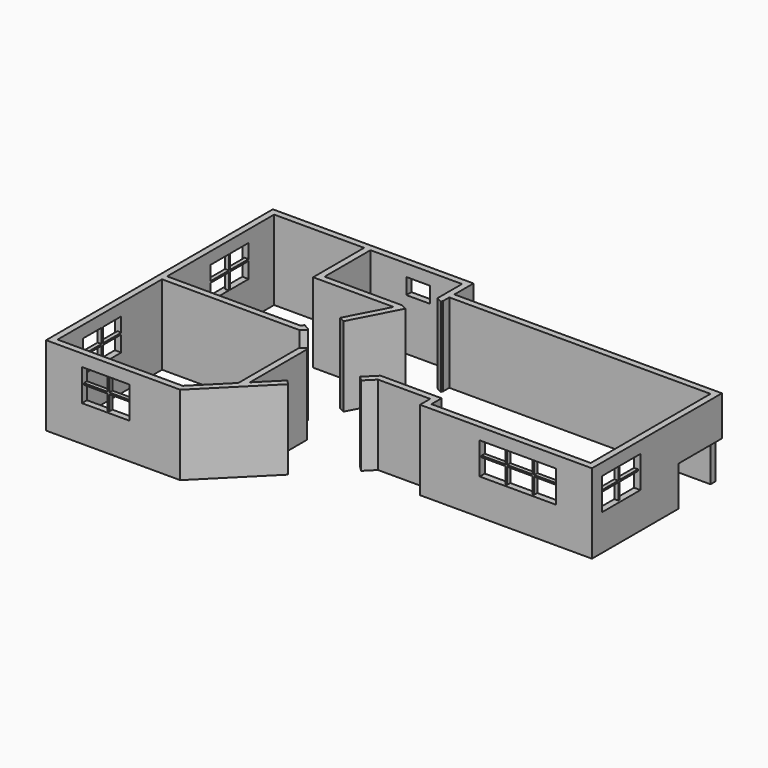
from build123d import *

# Parameters (mm, degrees)
F1_DEPTH  = 2540
F2_W      = 736.6
F2_H      = 457.2
F2_H_2    = 508
F3_DEPTH  = 203.2
F4_W      = 1524
F4_H      = 1016
F5_DEPTH  = 76.2
F6_W      = 762
F6_H      = 482.6
F6_W_2    = 711.2
F7_DEPTH  = 203.2
F8_W      = 1524
F8_H      = 1016
F9_DEPTH  = 76.2
F10_W     = 762
F10_H     = 457.2
F10_W_2   = 812.8
F10_H_2   = 508
F11_DEPTH = 203.2
F12_W     = 2438.4
F12_H     = 1016
F13_DEPTH = 76.2
F14_W     = 762
F14_H     = 508
F15_DEPTH = 203.2
F16_W     = 203.2
F16_H     = 1270
F16_W_2   = 1524
F17_DEPTH = 203.2
F18_W     = 736.6
F18_H     = 508
F19_DEPTH = 203.2
F20_W     = 1524
F20_H     = 1016
F21_DEPTH = 76.2


# Not quite as in the source:
# - ends of sketch curves that miss each other by under 0.0002 mm in the source are joined


with BuildPart() as f1:
    # F0 (on Top) → F1 (new body)
    with BuildSketch(Plane.XY):
        Polygon((0, 10668), (0, 1625.6), (4279.6544454742, 1625.6), (6192.0032212604, 3537.9487757862), (6048.3191233233, 3681.6328737233), (5385.1059684, 3018.4197188), (5385.1059684, 5299.2660923905), (5342.8269923446, 5354.1003717159), (5181.9059684, 5230.0251362632), (5181.9059684, 2815.2197188), (4195.4862496, 1828.8), (2071.3068791001, 1828.8), (203.2, 1828.8), (203.2, 5994.4), (4592.5486, 5994.4), (4753.4696239446, 6118.4752354526), (4696.3063146823, 6192.6139483473), (4516.9390764162, 6286.5061031958), (4470.4, 6197.6), (203.2, 6197.6), (203.2, 10464.8), (3073.4, 10464.8), (3073.4, 8432.8), (5640.4450235294, 8432.8), (4964.5662461846, 7141.6323844462), (5143.9334844506, 7047.7402295977), (5926.1799912072, 8542.1078451515), (5746.8127529412, 8636), (3276.6, 8636), (3276.6, 10464.8), (6197.6, 10464.8), (6197.6, 9702.8), (6197.6, 9497.163147027), (6194.4399227095, 9491.1262812504), (6373.8071609756, 9397.2341264019), (6400.8, 9448.8), (6400.8, 9702.8), (14732, 9702.8), (14732, 4927.6), (9652, 4927.6), (9652, 5334), (7700.6862496, 5334), (7341.4760047572, 4974.7897551572), (7485.1601026943, 4831.1056572201), (7784.8544454742, 5130.8), (9448.8, 5130.8), (9448.8, 4724.4), (14935.2, 4724.4), (14935.2, 9906), (6400.8, 9906), (6400.8, 10668), align=None)
    extrude(amount=F1_DEPTH)

    # F2 (on face) → F3 (cut)
    with BuildSketch(Plane(origin=(0, 0, 0), x_dir=(0, -1, 0), z_dir=(-1, 0, 0))):
        with Locations((-9080.5, 1930.4)):
            Rectangle(F2_W, F2_H)
        with Locations((-8293.1, 1930.4)):
            Rectangle(F2_W, F2_H)
        with Locations((-9080.5, 1397)):
            Rectangle(F2_W, F2_H_2)
        with Locations((-8293.1, 1397)):
            Rectangle(F2_W, F2_H_2)
        with Locations((-4000.5, 1930.4)):
            Rectangle(F2_W, F2_H)
        with Locations((-3213.1, 1930.4)):
            Rectangle(F2_W, F2_H)
        with Locations((-4000.5, 1397)):
            Rectangle(F2_W, F2_H_2)
        with Locations((-3213.1, 1397)):
            Rectangle(F2_W, F2_H_2)
    extrude(amount=-F3_DEPTH, mode=Mode.SUBTRACT)

    # F4 (on face) → F5 (cut)
    with BuildSketch(Plane(origin=(0, 0, 0), x_dir=(0, -1, 0), z_dir=(-1, 0, 0))):
        with Locations((-8686.8, 1651)):
            Rectangle(F4_W, F4_H)
        with Locations((-3606.8, 1651)):
            Rectangle(F4_W, F4_H)
    extrude(amount=-F5_DEPTH, mode=Mode.SUBTRACT)

    # F6 (on face) → F7 (cut)
    with BuildSketch(Plane.XZ.offset(-1625.6)):
        with Locations((1524, 1917.7)):
            Rectangle(F6_W, F6_H)
        with Locations((2311.4, 1917.7)):
            Rectangle(F6_W_2, F6_H)
        with Locations((1524, 1384.3)):
            Rectangle(F6_W, F6_H)
        with Locations((2311.4, 1384.3)):
            Rectangle(F6_W_2, F6_H)
    extrude(amount=-F7_DEPTH, mode=Mode.SUBTRACT)

    # F8 (on face) → F9 (cut)
    with BuildSketch(Plane.XZ.offset(-1625.6)):
        with Locations((1905, 1651)):
            Rectangle(F8_W, F8_H)
    extrude(amount=-F9_DEPTH, mode=Mode.SUBTRACT)

    # F10 (on face) → F11 (cut)
    with BuildSketch(Plane.XZ.offset(-4724.4)):
        with Locations((11734.8, 1930.4)):
            Rectangle(F10_W, F10_H)
        with Locations((12573, 1930.4)):
            Rectangle(F10_W_2, F10_H)
        with Locations((13411.2, 1930.4)):
            Rectangle(F10_W, F10_H)
        with Locations((11734.8, 1397)):
            Rectangle(F10_W, F10_H_2)
        with Locations((12573, 1397)):
            Rectangle(F10_W_2, F10_H_2)
        with Locations((13411.2, 1397)):
            Rectangle(F10_W, F10_H_2)
    extrude(amount=-F11_DEPTH, mode=Mode.SUBTRACT)

    # F12 (on face) → F13 (cut)
    with BuildSketch(Plane.XZ.offset(-4724.4)):
        with Locations((12573, 1651)):
            Rectangle(F12_W, F12_H)
    extrude(amount=-F13_DEPTH, mode=Mode.SUBTRACT)

    # F14 (on face) → F15 (cut)
    with BuildSketch(Plane(origin=(0, 10668, 0), x_dir=(-1, 0, 0), z_dir=(0, 1, 0))):
        with Locations((-4800.6, 1905)):
            Rectangle(F14_W, F14_H)
    extrude(amount=-F15_DEPTH, mode=Mode.SUBTRACT)

    # F16 (on face) → F17 (cut)
    with BuildSketch(Plane.YZ.offset(14935.2)):
        with Locations((9804.4, 635)):
            Rectangle(F16_W, F16_H)
        with Locations((8940.8, 635)):
            Rectangle(F16_W_2, F16_H)
    extrude(amount=-F17_DEPTH, mode=Mode.SUBTRACT)

    # F18 (on face) → F19 (cut)
    with BuildSketch(Plane.YZ.offset(14935.2)):
        Polygon((6654.8, 2159), (5130.8, 2159), (5130.8, 1701.8), (5867.4, 1701.8), (5867.4, 2155.3428173065), (5918.2, 2155.3428173065), (5918.2, 1701.8), (6654.8, 1701.8), align=None)
        with Locations((5499.1, 1397)):
            Rectangle(F18_W, F18_H)
        with Locations((6286.5, 1397)):
            Rectangle(F18_W, F18_H)
    extrude(amount=-F19_DEPTH, mode=Mode.SUBTRACT)

    # F20 (on face) → F21 (cut)
    with BuildSketch(Plane.YZ.offset(14935.2)):
        with Locations((5892.8, 1651)):
            Rectangle(F20_W, F20_H)
    extrude(amount=-F21_DEPTH, mode=Mode.SUBTRACT)


solid = f1.part
